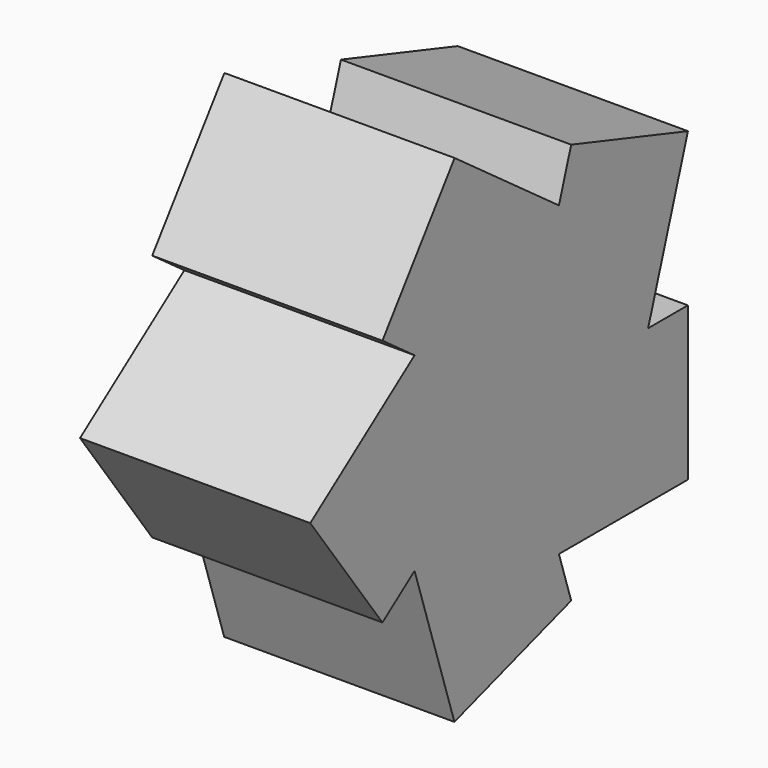
from build123d import *

# Parameters (mm, degrees)
F0_W     = 60
F0_H     = 55
F1_DEPTH = 40
F2_COUNT = 5


with BuildPart() as f1:
    # F0 (on Top) → F1 (new body)
    with BuildSketch(Plane.XY):
        with Locations((-30, 29.6852235304)):
            Rectangle(F0_W, F0_H)
    extrude(amount=F1_DEPTH)

    # F2: F1 ×5 about axis
    f2_axis = Axis((-30, 2.1852235304, 40), (-1, 0, 0))


with BuildPart() as f1_1:
    add(f1.part)
    for i in range(1, F2_COUNT):
        add(f1.part.rotate(f2_axis, i * 360 / F2_COUNT))


solid = f1_1.part
